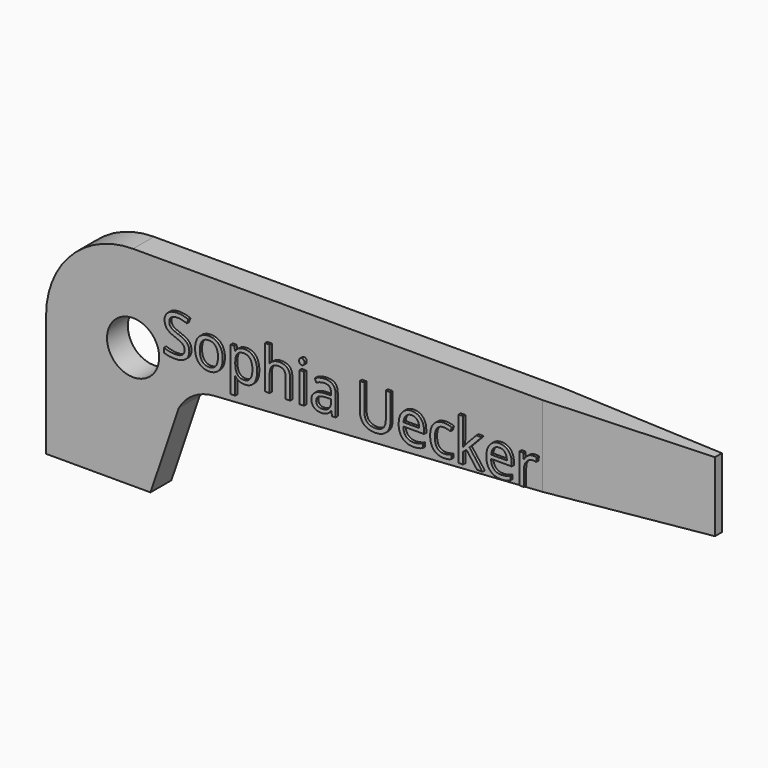
from build123d import *

# Parameters (mm, degrees)
F1_DEPTH     = 2.38125
F2_R         = 2.38125
F3_DEPTH     = 2.38225
F5_DEPTH     = 25.4
F6_TEXT_SIZE = 5.1194593353
F7_DEPTH     = 0.254


# Not quite as in the source:
# - Text() gives the source's letters only with a copy of the font that has no kerning and outlines rounded to 1/6400 em; it was checked with that copy


with BuildPart() as f1:
    # F0 (on Front) → F1 (new body)
    with BuildSketch(Plane.XZ):
        with BuildLine():
            Line((60.3885, 19.05), (7.9375, 19.05))
            ThreePointArc((7.9375, 19.05), (2.3248399243, 16.7251600757), (0, 11.1125))
            Line((0, 11.1125), (0, 0))
            Line((0, 0), (9.525, 0))
            Line((9.525, 0), (12.1103451907, 7.6262422093))
            ThreePointArc((12.1103451907, 7.6262422093), (13.4534811895, 9.0409189326), (15.3078989773, 9.6462776784))
            Line((15.3078989773, 9.6462776784), (60.3885, 12.7))
            Line((60.3885, 12.7), (60.3885, 19.05))
        make_face()
    extrude(amount=F1_DEPTH)

    # F2 (on face) → F3 (cut, through all)
    with BuildSketch(Plane.XZ.offset(2.38125)):
        with Locations((7.9375, 11.1125)):
            Circle(F2_R)
    extrude(amount=-F3_DEPTH, mode=Mode.SUBTRACT)

    # F4 (on face) → F5 (cut)
    with BuildSketch(Plane.XY.offset(19.05)):
        Polygon((60.3885, 0), (45.3009, 0), (60.3885, -0.79375), align=None)
        Polygon((60.3885, -2.38125), (60.3885, -1.5875), (45.3009, -2.38125), align=None)
    extrude(amount=-F5_DEPTH, mode=Mode.SUBTRACT)

    # F6 (on face) → F7 (join)
    with BuildSketch(Plane.XZ.offset(2.38125)):
        with Locations((10.7013540487, 11.6779785572)):
            Text('Sophia Uecker', F6_TEXT_SIZE, font='Open Sans', text_align=(TextAlign.LEFT, TextAlign.BOTTOM))
    extrude(amount=F7_DEPTH)


solid = f1.part
